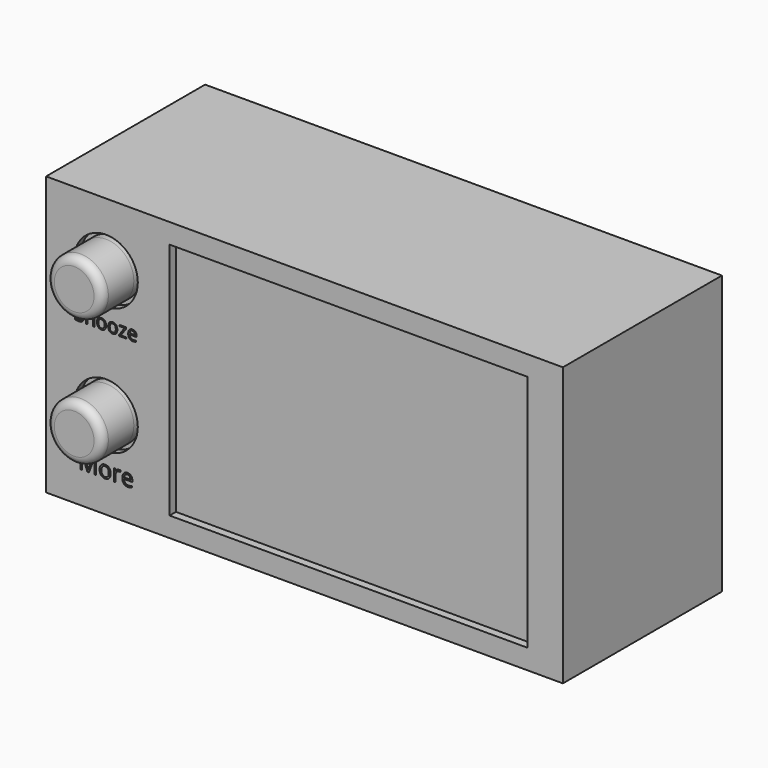
from build123d import *

# Parameters (mm, degrees)
F0_W           = 65
F0_H           = 35
F1_DEPTH       = 25
F2_W           = 45
F2_H           = 30
F3_DEPTH       = 1
F2_R           = 4
F2_R_2         = 3.5
F4_DEPTH       = 1
F5_DEPTH       = 5
F2_TEXT_SIZE   = 2.3445370455
F2_TEXT_SIZE_2 = 2.8126569563
F6_DEPTH       = 1
F7_R           = 1
F7_2_R         = 1
F8_DEPTH       = 0.5


# Not quite as in the source:
# - Text() gives the source's letters only with a copy of the font that has no kerning and outlines rounded to 1/6400 em; it was checked with that copy


with BuildPart() as f1:
    # F0 (on Front) → F1 (new body)
    with BuildSketch(Plane.XZ):
        Rectangle(F0_W, F0_H)
    extrude(amount=-F1_DEPTH)

    # F2 (on Front) → F3 (cut)
    with BuildSketch(Plane.XZ):
        with Locations((5.5357159674, 0)):
            Rectangle(F2_W, F2_H)
    extrude(amount=-F3_DEPTH, mode=Mode.SUBTRACT)

    # F2 (on Front) → F4 (cut)
    with BuildSketch(Plane.XZ):
        with Locations((-24.9642840326, 9.5)):
            Circle(F2_R)
        with Locations((-24.9642840326, 9.5)):
            Circle(F2_R_2, mode=Mode.SUBTRACT)
        with Locations((-24.9642840326, -6.5)):
            Circle(F2_R)
        with Locations((-24.9642840326, -6.5)):
            Circle(F2_R_2, mode=Mode.SUBTRACT)
    extrude(amount=-F4_DEPTH, mode=Mode.SUBTRACT)

    # F2 (on Front) → F6 (cut)
    with BuildSketch(Plane.XZ):
        with Locations((-28.9642840326, 2.8119333272)):
            Text('Snooze', F2_TEXT_SIZE, font='Open Sans', text_align=(TextAlign.LEFT, TextAlign.BOTTOM))
        with Locations((-28.4642840326, -13.5251130085)):
            Text('More', F2_TEXT_SIZE_2, font='Open Sans', text_align=(TextAlign.LEFT, TextAlign.BOTTOM))
    extrude(amount=-F6_DEPTH, mode=Mode.SUBTRACT)


with BuildPart() as f5:
    # F2 (on Front) → F5 (new body)
    with BuildSketch(Plane.XZ):
        with Locations((-24.9642840326, 9.5)):
            Circle(F2_R_2)
    extrude(amount=F5_DEPTH)

    # F7
    f7_edges = [f5.edges().sort_by_distance(p)[0] for p in [
        (-28.464284, -5, 9.5),
    ]]
    fillet(f7_edges, radius=F7_R)


with BuildPart() as f5b:
    # F2 (on Front) → F5, piece 2 (new body)
    with BuildSketch(Plane.XZ):
        with Locations((-24.9642840326, -6.5)):
            Circle(F2_R_2)
    extrude(amount=F5_DEPTH)

    # F7#2
    f7_2_edges = [f5b.edges().sort_by_distance(p)[0] for p in [
        (-28.464284, -5, -6.5),
    ]]
    fillet(f7_2_edges, radius=F7_2_R)


with BuildPart() as f8:
    # F2 (on Front) → F8 (new body)
    with BuildSketch(Plane.XZ):
        with Locations((5.5357159674, 0)):
            Rectangle(F2_W, F2_H)
    extrude(amount=-F8_DEPTH)


with BuildPart() as f8_1:
    # F9: moved
    add(f8.part.moved(Location((0, 0.5, 0))))


solid = Compound([f1.part, f5.part, f5b.part])
